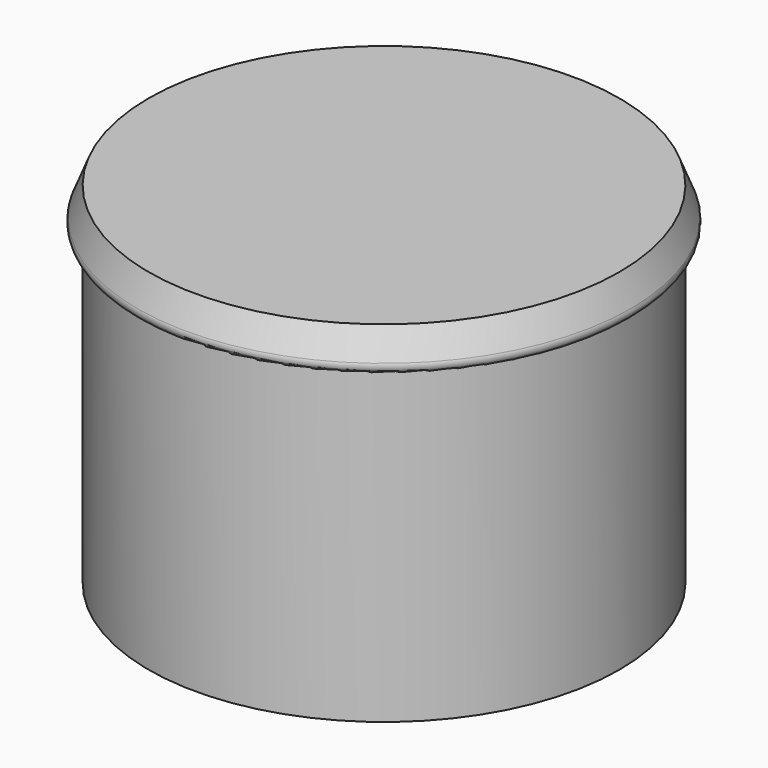
from build123d import *

# Parameters (mm, degrees)
F0_W    = 2
F0_H    = 5
F0_H_2  = 3
F3_SIZE = 1.99999
F5_R    = 1


# Not quite as in the source:
# - a fillet or chamfer that OpenCascade refuses, or shapes differently, is made with other operations: its cross-section is extruded or revolved along the edge and cut away or added
# - a fillet or chamfer is up to 0.001 mm smaller than in the source, because OpenCascade refuses the exact size


with BuildPart() as f1:
    # F0 (on Front) → F1 (revolve)
    with BuildSketch(Plane.XZ):
        Polygon((30, 0), (27, 0), (27, -3), (27, -6), (27, -11), (27, -14), (27, -19), (27, -22), (27, -25), (27, -39.6280139685), (30, -39.6280139685), align=None)
    revolve(axis=Axis((0, 0, -12.5), (0, 0, -1)))


with BuildPart() as f2:
    # F0 (on Front) → F2 (revolve)
    with BuildSketch(Plane.XZ):
        Polygon((0, 5), (0, 0), (22, 0), (25, 0), (27, 0), (30, 0), (30, 5), align=None)
        with Locations((31, 2.5)):
            Rectangle(F0_W, F0_H)
        Polygon((25, 0), (22, 0), (22, -25), (25, -25), (25, -22), (25, -19), (25, -14), (25, -11), (25, -6), (25, -3), align=None)
        with Locations((26, -1.5)):
            Rectangle(F0_W, F0_H_2)
        with Locations((26, -8.5)):
            Rectangle(F0_W, F0_H)
        with Locations((26, -16.5)):
            Rectangle(F0_W, F0_H)
        with Locations((26, -23.5)):
            Rectangle(F0_W, F0_H_2)
    revolve(axis=Axis((0, 0, -12.5), (0, 0, -1)))

    # F3 (size 2 in the source; OpenCascade refuses exactly that, so slightly less here)
    f3_edges = [f2.edges().sort_by_distance(p)[0] for p in [
        (-27, 0, -22),
        (-27, 0, -19),
        (-27, 0, -14),
        (-27, 0, -6),
        (-27, 0, -11),
        (-27, 0, -3),
    ]]
    chamfer(f3_edges, length=F3_SIZE)

    # F4: chamfer of 2 x 5 on 1 edges, made by hand

    # F4_s1 → F4_t2 (revolve, cut)
    with BuildSketch(Plane.XZ):
        Polygon((32, 0), (30, 5), (32, 5), align=None)
    revolve(axis=Axis((0, 0, 5), (0, 0, -1)), mode=Mode.SUBTRACT)

    # F5
    f5_edges = [f2.edges().sort_by_distance(p)[0] for p in [
        (-32, 0, 0),
    ]]
    fillet(f5_edges, radius=F5_R)


solid = Compound([f1.part, f2.part])
